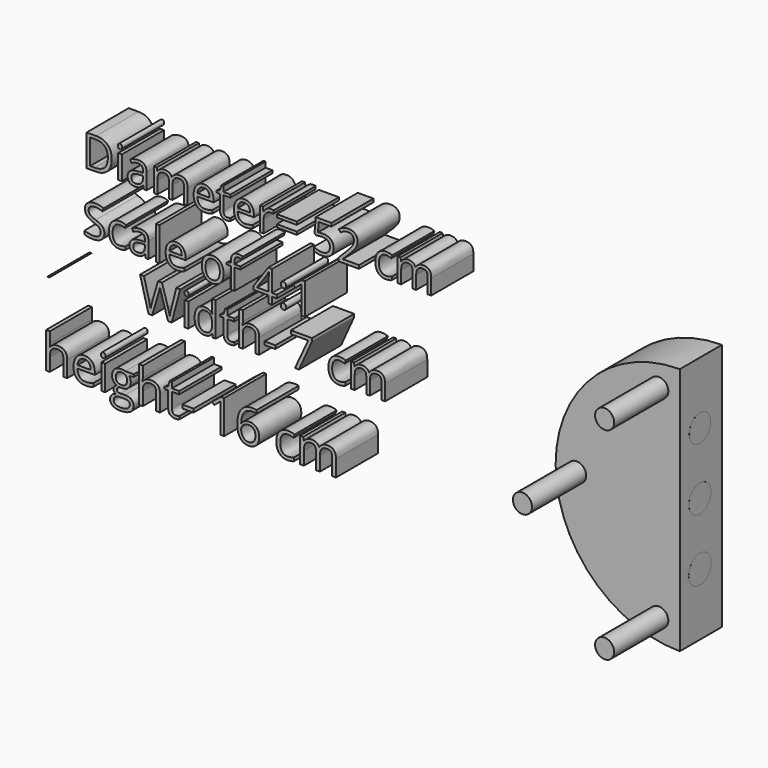
from build123d import *

# Parameters (mm, degrees)
F0_TEXT_SIZE   = 58.6420550842
F0_TEXT_SIZE_2 = 0.4119498448
F0_TEXT_SIZE_3 = 59.4275589618
F0_TEXT_SIZE_4 = 62.5022169616
F1_DEPTH       = 70
F2_R           = 12.7
F3_DEPTH       = 90
F5_DEPTH       = 0.0254


# Not quite as in the source:
# - Text() gives the source's letters only with a copy of the font that has no kerning and outlines rounded to 1/6400 em; it was checked with that copy


with BuildPart() as f1:
    # F0 (on Front) → F1 (new body)
    with BuildSketch(Plane.XZ):
        with BuildLine():
            Line((0, -165.1), (0, 165.1))
            ThreePointArc((0, 165.1), (-165.1, 0), (0, -165.1))
        make_face()
        with Locations((-794.3927826536, 143.7842250549)):
            Text('Diameter= 52 cm', F0_TEXT_SIZE, font='Open Sans', text_align=(TextAlign.LEFT, TextAlign.BOTTOM))
        with Locations((-794.3927826536, 64.0310301403)):
            Text('Scale of 4:1', F0_TEXT_SIZE, font='Open Sans', text_align=(TextAlign.LEFT, TextAlign.BOTTOM))
        with Locations((-840.6738908258, -0.2966038883)):
            Text('Width= 6 cm', F0_TEXT_SIZE_2, font='Open Sans', text_align=(TextAlign.LEFT, TextAlign.BOTTOM))
        with Locations((-718.3661319003, 0)):
            Text('Width- 7 cm', F0_TEXT_SIZE_3, font='Open Sans', text_align=(TextAlign.LEFT, TextAlign.BOTTOM))
        with Locations((-847.8638529778, -110.4172617197)):
            Text('height- 16 cm', F0_TEXT_SIZE_4, font='Open Sans', text_align=(TextAlign.LEFT, TextAlign.BOTTOM))
    extrude(amount=F1_DEPTH)

    # F2 (on face) → F3 (join)
    with BuildSketch(Plane.XZ.offset(70)):
        with Locations((-27.94, 134.2841092609)):
            Circle(F2_R)
        with Locations((-27.94, -134.2841092609)):
            Circle(F2_R)
        with Locations((-137.16, 0)):
            Circle(F2_R)
    extrude(amount=F3_DEPTH)

    # F4 (on face) → F5 (join)
    with BuildSketch(Plane.YZ):
        with BuildLine():
            Line((-36.5225747228, 18.3944704189), (-36.5225747228, 0))
            Line((-36.5225747228, 0), (-36.5225747228, -18.3944704189))
            ThreePointArc((-36.5225747228, -18.3944704189), (-23.5157199532, -13.0068547695), (-18.1281043039, 0))
            ThreePointArc((-18.1281043039, 0), (-23.5157199532, 13.0068547695), (-36.5225747228, 18.3944704189))
        make_face()
        with BuildLine():
            Line((-36.5225747228, -18.3944704189), (-36.5225747228, 0))
            Line((-36.5225747228, 0), (-36.5225747228, 18.3944704189))
            ThreePointArc((-36.5225747228, 18.3944704189), (-54.9170451416, 0), (-36.5225747228, -18.3944704189))
        make_face()
        with BuildLine():
            ThreePointArc((-17.8029992731, -82.55), (-23.2858359814, -69.3132612586), (-36.5225747228, -63.8304245503))
            Line((-36.5225747228, -63.8304245503), (-36.5225747228, -101.2695754497))
            ThreePointArc((-36.5225747228, -101.2695754497), (-23.2858359814, -95.7867387414), (-17.8029992731, -82.55))
        make_face()
        with BuildLine():
            Line((-36.5225747228, -101.2695754497), (-36.5225747228, -63.8304245503))
            ThreePointArc((-36.5225747228, -63.8304245503), (-55.2421501724, -82.55), (-36.5225747228, -101.2695754497))
        make_face()
        with BuildLine():
            ThreePointArc((-36.5225747228, 100.3705031784), (-54.3430779012, 82.55), (-36.5225747228, 64.7294968216))
            Line((-36.5225747228, 64.7294968216), (-36.5225747228, 100.3705031784))
        make_face()
        with BuildLine():
            Line((-36.5225747228, 100.3705031784), (-36.5225747228, 64.7294968216))
            ThreePointArc((-36.5225747228, 64.7294968216), (-23.9215760811, 69.9490013584), (-18.7020715443, 82.55))
            ThreePointArc((-18.7020715443, 82.55), (-23.9215760811, 95.1509986416), (-36.5225747228, 100.3705031784))
        make_face()
    extrude(amount=F5_DEPTH)


solid = f1.part
